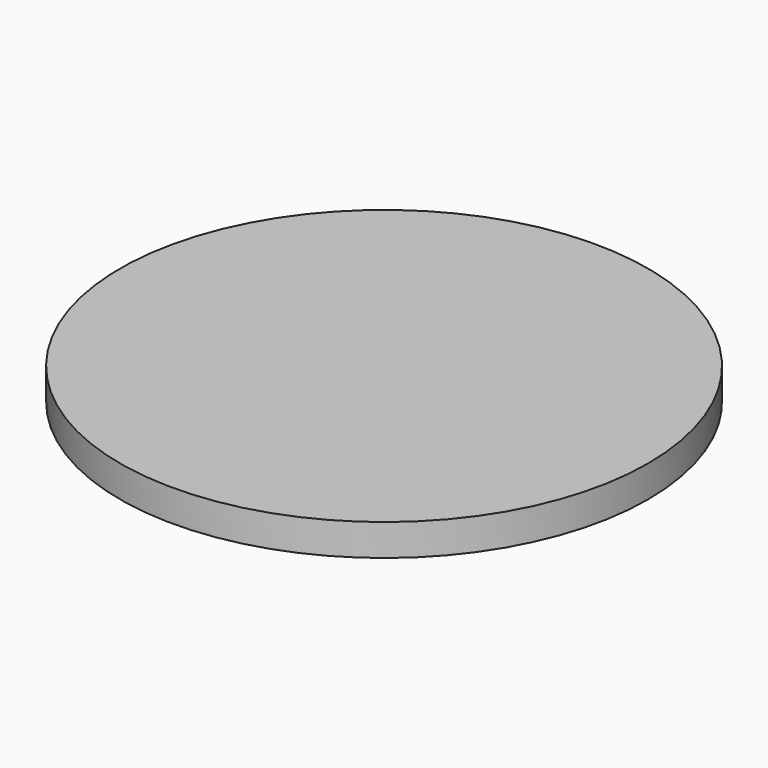
from build123d import *

# Parameters (mm, degrees)
F1_R     = 52.9171357006
F2_DEPTH = 6.35


# Not quite as in the source:
# - a variable given as a bare number and used for a length is read in inches; the dataset says mm whatever the document's units were


with BuildPart() as f2:
    # F1 (on Top) → F2 (new body)
    with BuildSketch(Plane.XY):
        Circle(F1_R)
    extrude(amount=F2_DEPTH)


solid = f2.part
